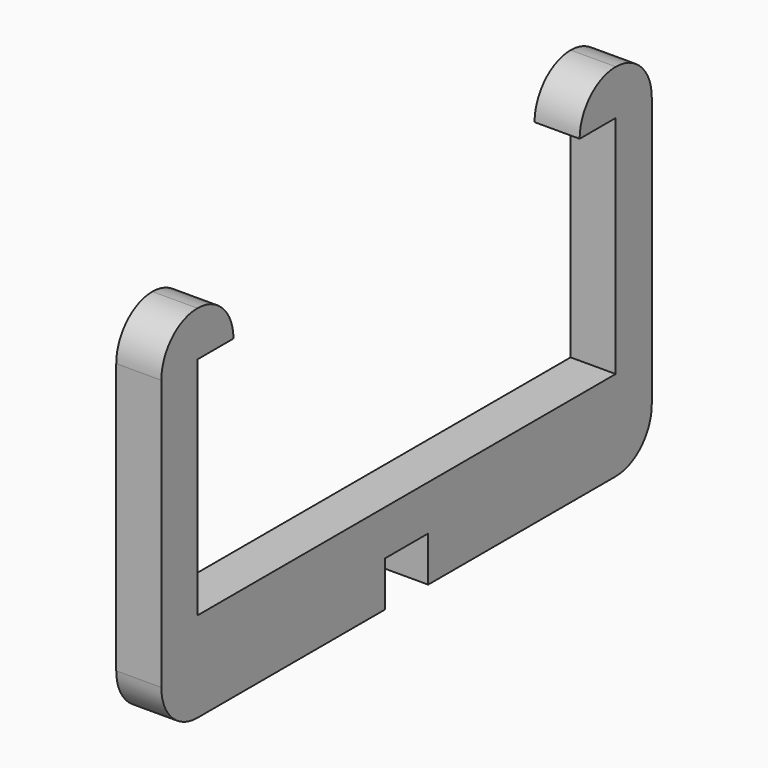
from build123d import *

# Parameters (mm, degrees)
F0_W     = 5
F0_H     = 68
F1_DEPTH = 10
F2_W     = 5
F2_H     = 5
F3_DEPTH = 30
F5_W     = 5
F5_H     = 5
F6_DEPTH = 5
F4_W     = 5
F4_H     = 5
F7_DEPTH = 5
F8_W     = 5
F8_H     = 6
F9_DEPTH = 5
F10_R    = 4.99999
F11_R    = 5


# Not quite as in the source:
# - a fillet or chamfer is up to 0.001 mm smaller than in the source, because OpenCascade refuses the exact size


with BuildPart() as f1:
    # F0 (on Top) → F1 (new body)
    with BuildSketch(Plane.XY):
        Rectangle(F0_W, F0_H)
    extrude(amount=F1_DEPTH)

    # F2 (on face) → F3 (join)
    with BuildSketch(Plane.XY.offset(10)):
        with Locations((0, 31.5)):
            Rectangle(F2_W, F2_H)
        with Locations((0, -31.5)):
            Rectangle(F2_W, F2_H)
    extrude(amount=F3_DEPTH)

    # F5 (on face) → F6 (join)
    with BuildSketch(Plane(origin=(0, -29, 0), x_dir=(-1, 0, 0), z_dir=(0, 1, 0))):
        with Locations((0, 37.5)):
            Rectangle(F5_W, F5_H)
    extrude(amount=F6_DEPTH)

    # F4 (on face) → F7 (join)
    with BuildSketch(Plane.XZ.offset(-29)):
        with Locations((0, 37.5)):
            Rectangle(F4_W, F4_H)
    extrude(amount=F7_DEPTH)

    # F8 (on face) → F9 (cut)
    with BuildSketch(Plane(origin=(0, 0, 0), x_dir=(1, 0, 0), z_dir=(0, 0, -1))):
        Rectangle(F8_W, F8_H)
    extrude(amount=-F9_DEPTH, mode=Mode.SUBTRACT)

    # F10 (radius 5 in the source; OpenCascade refuses exactly that, so slightly less here)
    f10_edges = [f1.edges().sort_by_distance(p)[0] for p in [
        (0, 24, 40),
        (0, -24, 40),
        (0, -34, 40),
    ]]
    fillet(f10_edges, radius=F10_R)

    # F11
    f11_edges = [f1.edges().sort_by_distance(p)[0] for p in [
        (0, 34, 40),
        (0, 34, 0),
        (0, -34, 0),
    ]]
    fillet(f11_edges, radius=F11_R)


solid = f1.part
